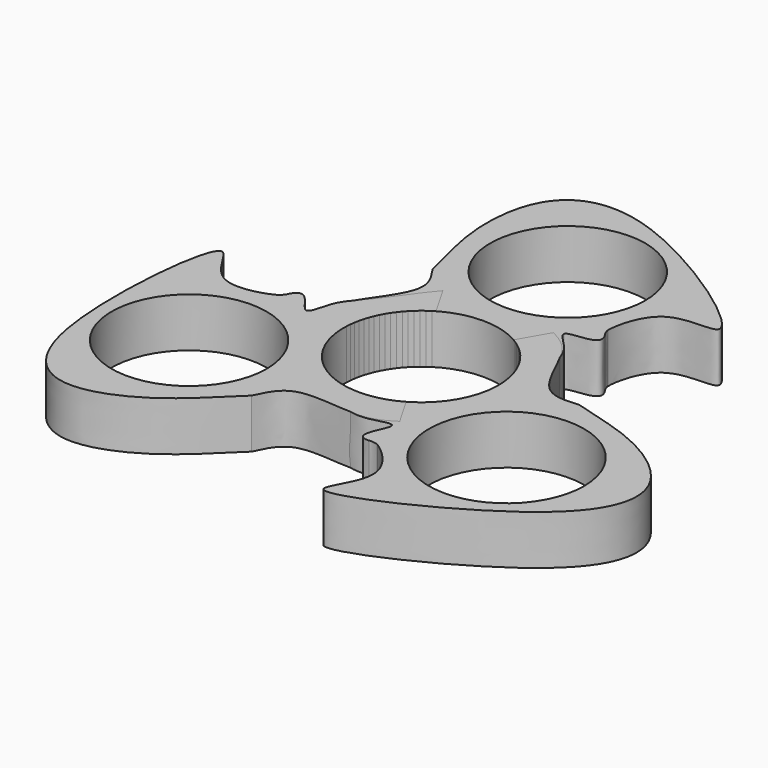
from build123d import *

# Parameters (mm, degrees)
F0_R     = 11
F1_DEPTH = 7
F3_F1_R  = 0.1562073455
F4_COUNT = 3


with BuildPart() as f1:
    # F0 (on Top) → F1 (new body)
    with BuildSketch(Plane.XY):
        with BuildLine():
            ThreePointArc((-11, 0), (0, 11), (11, 0))
            Line((11, 0), (15.9760136157, 0))
            add(Edge.make_bspline(
                [(12.7080408856, 16.6851170361), (14.2245192131, 14.383231597), (6.616117108, 15.2541256327), (11.7787673039, 11.5296924988), (12.3970789149, 7.6736957262), (15.0250841653, 2.8049501499), (15.9760136157, 0)],
                knots=[0, 0, 0, 0, 0.2328471326, 0.4311179611, 0.6703855557, 1, 1, 1, 1], degree=3))
            add(Edge.make_bspline(
                [(12.2105782685, 17.8332442257), (12.2095235298, 17.4766927528), (12.2919432041, 16.76906879), (12.557796057, 16.7301087153), (12.7080408856, 16.6851170361)],
                knots=[0.943264963, 0.943264963, 0.943264963, 0.943264963, 0.9659751094, 1, 1, 1, 1], degree=3))
            add(Edge.make_bspline(
                [(12.2105782685, 17.8332442257), (12.2085319919, 17.8591208489), (12.2086199114, 17.8821246392), (12.2111852957, 17.9015738893)],
                knots=[0.8716103238, 0.8716103238, 0.8716103238, 0.8716103238, 0.9382173807, 0.9382173807, 0.9382173807, 0.9382173807], degree=3))
            add(Edge.make_bspline(
                [(-12.1004805482, 17.1632855393), (-12.9164125838, 20.7040955058), (-15.0334520238, 27.0999034766), (-13.6017674423, 39.9554067289), (-0.4004001164, 43.5633067225), (29.115658469, 22.7742261561), (13.9244510473, 26.7031215449), (12.2364707444, 19.6240449582), (12.2111852957, 17.9015738893)],
                knots=[0, 0, 0, 0, 0.1534795768, 0.3080574381, 0.4727247205, 0.7124592697, 0.834855538, 0.9418326275, 0.9418326275, 0.9418326275, 0.9418326275], degree=3))
            add(Edge.make_bspline(
                [(-12.1004805482, 17.1632855393), (-11.0967010634, 15.7449317326), (-8.7147440055, 12.3792474763), (-15.8903695152, 4.7262210134), (-15.7801721676, 1.3776649819), (-15.735, 0)],
                knots=[0, 0, 0, 0, 0.3000596392, 0.7120278226, 1, 1, 1, 1], degree=3))
            Line((-15.735, 0), (-11, 0))
        make_face()
        with Locations((0, 26)):
            Circle(F0_R, mode=Mode.SUBTRACT)
        with BuildLine():
            add(Edge.make_bspline(
                [(12.2105782685, 17.8332442257), (12.2095235298, 17.4766927528), (12.2919432041, 16.76906879), (12.557796057, 16.7301087153), (12.7080408856, 16.6851170361)],
                knots=[0.943264963, 0.943264963, 0.943264963, 0.943264963, 0.9659751094, 1, 1, 1, 1], degree=3))
            add(Edge.make_bspline(
                [(12.7080408856, 16.6851170361), (12.6234894791, 16.772823048), (12.4453669865, 17.0541620514), (12.2247788455, 17.6536678295), (12.2105782685, 17.8332442257)],
                knots=[0, 0, 0, 0, 0.4093763173, 0.8716103238, 0.8716103238, 0.8716103238, 0.8716103238], degree=3))
        make_face()
    extrude(amount=F1_DEPTH)

    # F3: fillet of radius 0.1562073455 on 1 edges, made by hand

    # F3_f1
    f3_f1_edges = [f1.edges().sort_by_distance(p)[0] for p in [
        (12.2111852957, 17.9015738893, 3.5),
    ]]
    fillet(f3_f1_edges, radius=F3_F1_R)


with BuildPart() as f4_1:
    # F4: instance of F1
    add(f1.part.rotate(Axis((0, 0, 6.8635325879), (0, 0, -1)), 1 * 360 / F4_COUNT))


with BuildPart() as f4_2:
    # F4: instance of F1
    add(f1.part.rotate(Axis((0, 0, 6.8635325879), (0, 0, -1)), 2 * 360 / F4_COUNT))


solid = Compound([f1.part, f4_1.part, f4_2.part])
